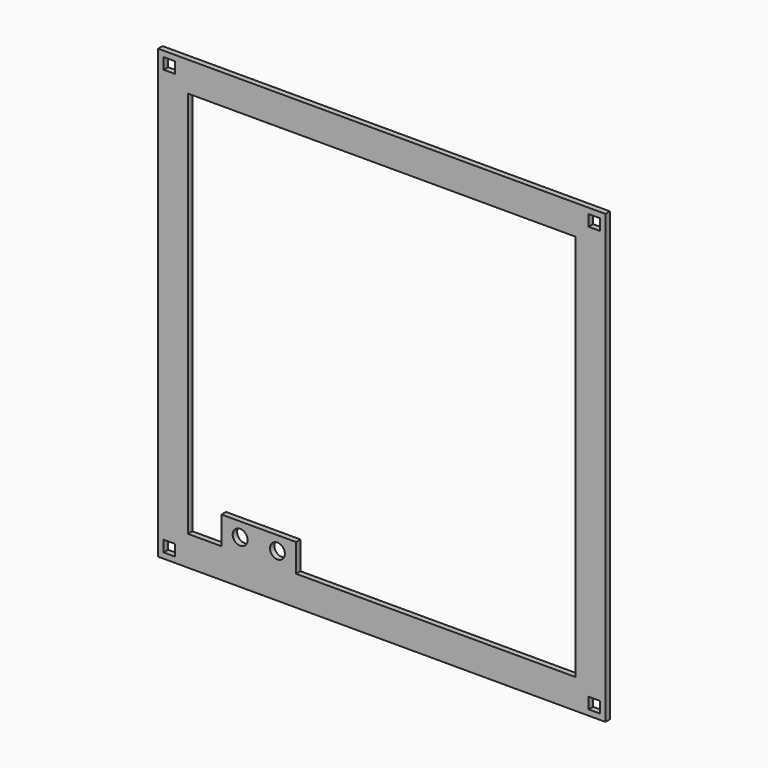
from build123d import *

# Parameters (mm, degrees)
F1_W     = 240
F1_H     = 240
F1_W_2   = 6
F1_H_2   = 6
F1_W_3   = 208
F1_H_3   = 208
F2_DEPTH = 3
F3_DEPTH = 25
F8_W     = 40
F8_H     = 15
F8_R     = 4
F9_DEPTH = 3


with BuildPart() as f2:
    # F1 (on Front) → F2 (new body)
    with BuildSketch(Plane.XZ):
        with Locations((120, 120)):
            Rectangle(F1_W, F1_H)
        with Locations((6, 234)):
            Rectangle(F1_W_2, F1_H_2, mode=Mode.SUBTRACT)
        with Locations((120, 120)):
            Rectangle(F1_W_3, F1_H_3, mode=Mode.SUBTRACT)
        with Locations((6, 234)):
            Rectangle(F1_W_2, F1_H_2)
    extrude(amount=F2_DEPTH)

    # F1 (on Front) → F3 (cut)
    with BuildSketch(Plane.XZ):
        with Locations((6, 234)):
            Rectangle(F1_W_2, F1_H_2)
    extrude(amount=F3_DEPTH, mode=Mode.SUBTRACT)

    # F5: F2 across plane


with BuildPart() as f2_1:
    add(f2.part)
    add(f2.part.mirror(Plane(origin=(120, -1.5, 120), x_dir=(0, -1, 0), z_dir=(-1, 0, 0))), mode=Mode.INTERSECT)

    # F7: F2 across plane


with BuildPart() as f2_2:
    add(f2_1.part)
    add(f2_1.part.mirror(Plane(origin=(120, -1.5, 120), x_dir=(1, 0, 0), z_dir=(0, 0, 1))), mode=Mode.INTERSECT)

    # F8 (on face) → F9 (join)
    with BuildSketch(Plane.XZ.offset(3)):
        with Locations((54, 23.5)):
            Rectangle(F8_W, F8_H)
        with Locations((44, 23.5)):
            Circle(F8_R, mode=Mode.SUBTRACT)
        with Locations((64, 23.5)):
            Circle(F8_R, mode=Mode.SUBTRACT)
    extrude(amount=-F9_DEPTH)


solid = f2_2.part
